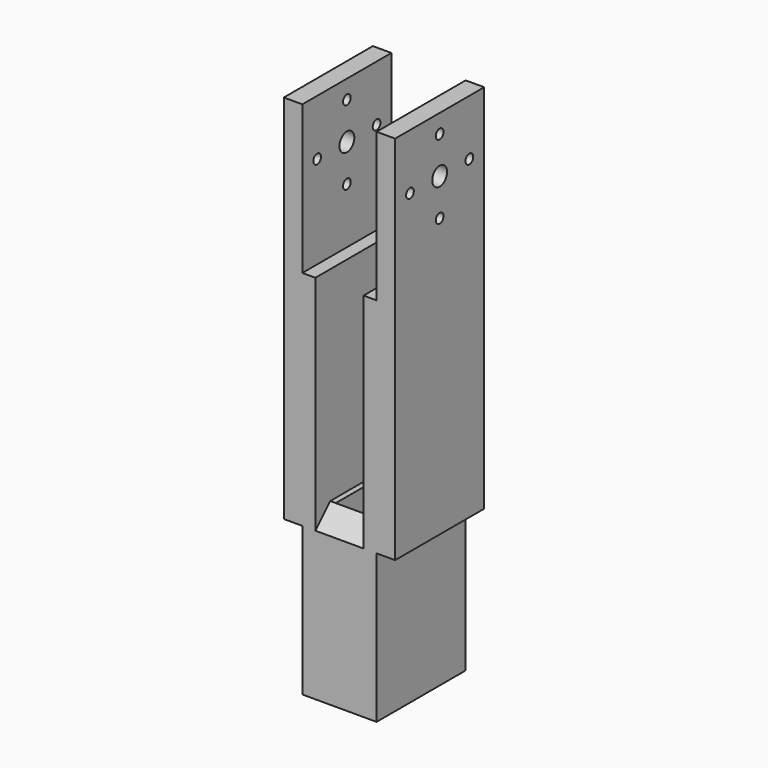
from build123d import *

# Parameters (mm, degrees)
F1_DEPTH = 6.35
F2_DEPTH = 76.2
F0_W     = 6.35
F0_H     = 38.1
F3_DEPTH = 127
F5_D     = 6.35
F6_SIZE  = 6.34999
F7_D     = 3.302
F8_DEPTH = 50.8


# Not quite as in the source:
# - a fillet or chamfer is up to 0.001 mm smaller than in the source, because OpenCascade refuses the exact size


with BuildPart() as f1:
    # F0 (on Top) → F1 (new body)
    with BuildSketch(Plane.XY):
        Polygon((-6.35, -12.7), (-6.35, 12.7), (-8.255, 12.7), (-8.255, -19.05), (8.255, -19.05), (8.255, 12.7), (6.35, 12.7), (6.35, -12.7), align=None)
    extrude(amount=F1_DEPTH)

    # F0 (on Top) → F2 (join)
    with BuildSketch(Plane.XY):
        Polygon((-8.255, -19.05), (-8.255, 12.7), (-8.255, 19.05), (-12.7, 19.05), (-12.7, -19.05), align=None)
        Polygon((8.255, 19.05), (8.255, 12.7), (8.255, -19.05), (12.7, -19.05), (12.7, 19.05), align=None)
        Polygon((-8.255, 12.7), (-6.35, 12.7), (6.35, 12.7), (8.255, 12.7), (8.255, 19.05), (-8.255, 19.05), align=None)
    extrude(amount=F2_DEPTH)

    # F0 (on Top) → F3 (join)
    with BuildSketch(Plane.XY):
        with Locations((-15.875, 0)):
            Rectangle(F0_W, F0_H)
        with Locations((15.875, 0)):
            Rectangle(F0_W, F0_H)
    extrude(amount=F3_DEPTH)

    # F5 (through all)
    with Locations(Plane.YZ.offset(19.05)):
        with Locations((0, 107.95)):
            Hole(F5_D / 2)

    # F6 (size 6.35 in the source; OpenCascade refuses exactly that, so slightly less here)
    f6_edges = [f1.edges().sort_by_distance(p)[0] for p in [
        (0, -19.05, 6.35),
    ]]
    chamfer(f6_edges, length=F6_SIZE)

    # F7 (through all)
    with Locations(Plane.YZ.offset(19.05)):
        with Locations((0, 120.65), (0, 95.25), (12.7, 107.95), (-12.7, 107.95)):
            Hole(F7_D / 2)

    # F0 (on Top) → F8 (join)
    with BuildSketch(Plane.XY):
        Polygon((-8.255, 12.7), (-6.35, 12.7), (6.35, 12.7), (8.255, 12.7), (8.255, 19.05), (-8.255, 19.05), align=None)
        Polygon((-8.255, -19.05), (-8.255, 12.7), (-8.255, 19.05), (-12.7, 19.05), (-12.7, -19.05), align=None)
        Polygon((-6.35, -12.7), (-6.35, 12.7), (-8.255, 12.7), (-8.255, -19.05), (8.255, -19.05), (8.255, 12.7), (6.35, 12.7), (6.35, -12.7), align=None)
        Polygon((8.255, 19.05), (8.255, 12.7), (8.255, -19.05), (12.7, -19.05), (12.7, 19.05), align=None)
    extrude(amount=-F8_DEPTH)


solid = f1.part
